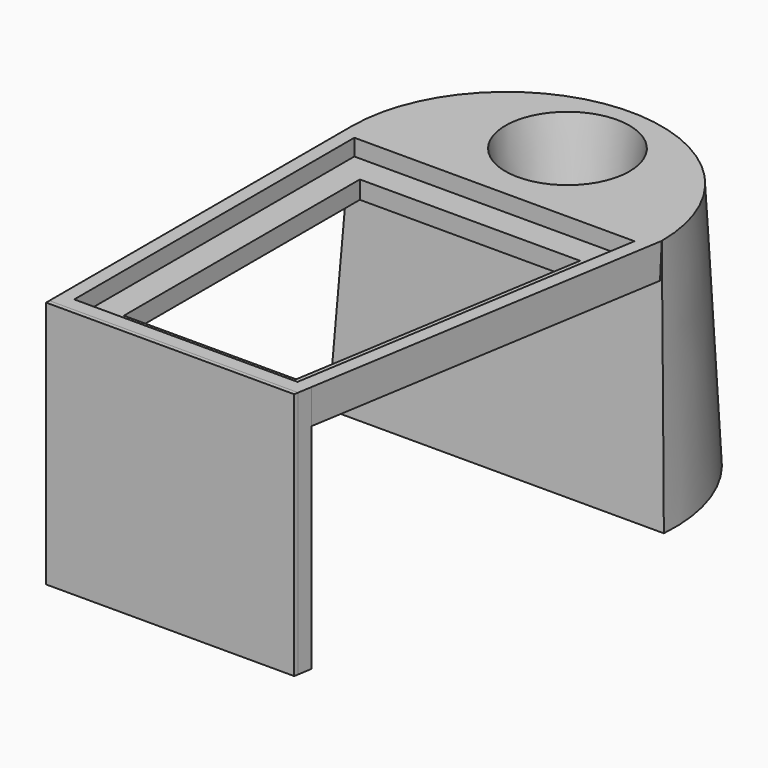
from build123d import *

# Parameters (mm, degrees)
F1_DEPTH               = 180
F2_DEPTH               = 180
F3_DEPTH               = 25
F0_R                   = 45
F4_DEPTH               = 180
DRAFT_F4_DRAFTED_ANGLE = -3
F5_START               = -12
F5_DEPTH               = 13
F6_DEPTH               = 100
F6_TAPER               = 8


# Not quite as in the source:
# - an extrude with a draft is written as a straight extrude whose walls are then drafted


with BuildPart() as f1:
    # F0 (on Top) → F1 (new body)
    with BuildSketch(Plane.XY):
        Polygon((-80.1345139742, 0.6964678168), (-80.1345139742, -2.3035321832), (99.8654860258, -2.3035321832), (100.3528506467, 0.6964678168), align=None)
    extrude(amount=-F1_DEPTH)


with BuildPart() as f2:
    # F0 (on Top) → F2 (new body)
    with BuildSketch(Plane.XY):
        Polygon((-80.1345139742, 10.6964705363), (-80.1345139742, 0.6964678168), (100.3528506467, 0.6964678168), (101.977399825, 10.6964705363), (91.846298482, 10.6964705363), (-70.1345112547, 10.6964705363), align=None)
    extrude(amount=-F2_DEPTH)

    # F0 (on Top) → F3 (join)
    with BuildSketch(Plane.XY):
        Polygon((-80.1345139742, 274.6964678168), (-80.1345139742, 10.6964705363), (-70.1345112547, 10.6964705363), (-70.1345112547, 264.6964650974), (133.1098355046, 264.6964650974), (91.846298482, 10.6964705363), (101.977399825, 10.6964705363), (144.8654860258, 274.6964678168), align=None)
    extrude(amount=-F3_DEPTH)


with BuildPart() as f4_drafted:
    # F0 (on Top) → F4 (new body)
    with BuildSketch(Plane.XY):
        with BuildLine():
            ThreePointArc((144.8654860258, 274.6964678168), (32.3654860258, 387.1964678168), (-80.1345139742, 274.6964678168))
            Line((-80.1345139742, 274.6964678168), (144.8654860258, 274.6964678168))
        make_face()
        with Locations((32.3654860258, 329.8269510269)):
            Circle(F0_R, mode=Mode.SUBTRACT)
        with Locations((32.3654860258, 329.8269510269)):
            Circle(F0_R)
    extrude(amount=-F4_DEPTH)

    # draft_F4_drafted
    draft_f4_drafted_walls = [f4_drafted.faces().sort_by_distance(p)[0] for p in [
        (32.3654860258, 274.6964678168, -120),
        (32.3654860258, 387.1964678168, -120),
    ]]
    draft(draft_f4_drafted_walls, neutral_plane=Plane(origin=(0, 0, 0), x_dir=(1, 0, 0), z_dir=(0, 0, -1)), angle=DRAFT_F4_DRAFTED_ANGLE)


with BuildPart() as f2_1:
    add(f2.part)

    # join_F4_drafted: union F4_drafted
    add(f4_drafted.part)

    # F0 (on Top) → F5 (join)
    with BuildSketch(Plane.XY.offset(F5_START)):
        Polygon((-70.1345112547, 264.6964650974), (-70.1345112547, 10.6964705363), (91.846298482, 10.6964705363), (133.1098355046, 264.6964650974), align=None)
        Polygon((74.8331991595, 30.6964700893), (-50.1345117018, 30.6964700893), (-50.1345117018, 244.6964655444), (109.5985413814, 244.6964655444), align=None, mode=Mode.SUBTRACT)
    extrude(amount=-F5_DEPTH)

    # F0 (on Top) → F6 (cut)
    with BuildSketch(Plane.XY):
        with Locations((32.3654860258, 329.8269510269)):
            Circle(F0_R)
    extrude(amount=-F6_DEPTH, taper=F6_TAPER, mode=Mode.SUBTRACT)


solid = Compound([f1.part, f2_1.part])
